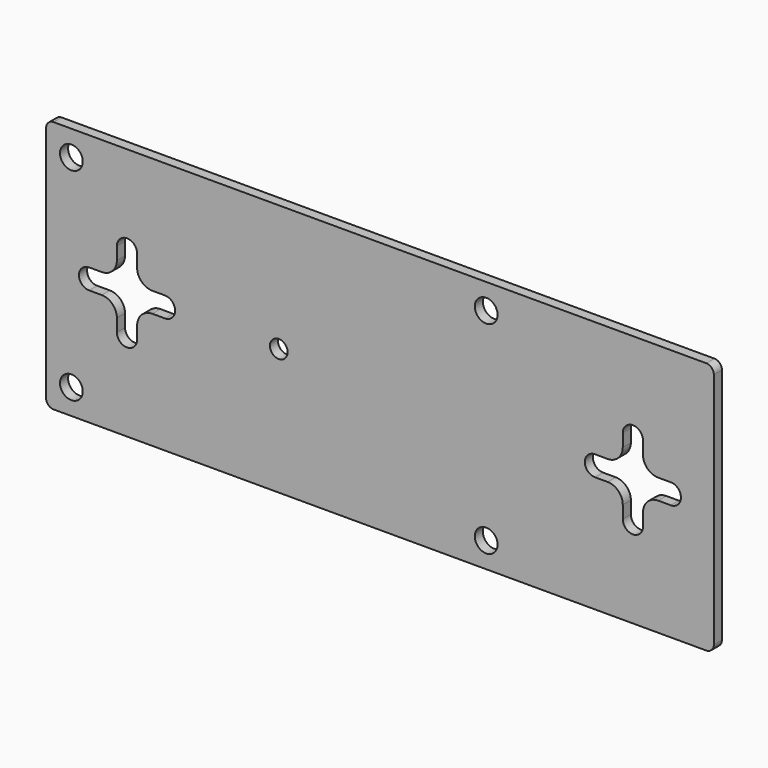
from build123d import *

# Parameters (mm, degrees)
F0_W     = 92
F0_H     = 50
F0_R     = 2.25
F0_R_2   = 1.75
F0_W_2   = 40
F1_DEPTH = 2
F2_R     = 3
F3_R     = 1.5


# Not quite as in the source:
# - a feature names something its author has since deleted; it is built from what else it names


with BuildPart() as f1:
    # F0 (on Front) → F1 (new body)
    with BuildSketch(Plane.XZ):
        with Locations((46, 25)):
            Rectangle(F0_W, F0_H)
        with Locations((5, 5)):
            Circle(F0_R, mode=Mode.SUBTRACT)
        with Locations((87, 5)):
            Circle(F0_R, mode=Mode.SUBTRACT)
        with BuildLine():
            Line((8.5, 27), (14, 27))
            Line((14, 27), (14, 32.5))
            ThreePointArc((14, 32.5), (16, 34.5), (18, 32.5))
            Line((18, 32.5), (18, 27))
            Line((18, 27), (23.5, 27))
            ThreePointArc((23.5, 27), (25.5, 25), (23.5, 23))
            Line((23.5, 23), (18, 23))
            Line((18, 23), (18, 17.5))
            ThreePointArc((18, 17.5), (16, 15.5), (14, 17.5))
            Line((14, 17.5), (14, 23))
            Line((14, 23), (8.5, 23))
            ThreePointArc((8.5, 23), (6.5, 25), (8.5, 27))
        make_face(mode=Mode.SUBTRACT)
        with Locations((46, 25)):
            Circle(F0_R_2, mode=Mode.SUBTRACT)
        with Locations((5, 45)):
            Circle(F0_R, mode=Mode.SUBTRACT)
        with Locations((87, 45)):
            Circle(F0_R, mode=Mode.SUBTRACT)
        with Locations((112, 25)):
            Rectangle(F0_W_2, F0_H)
        with BuildLine():
            Line((114, 27), (114, 32.5))
            ThreePointArc((114, 32.5), (116, 34.5), (118, 32.5))
            Line((118, 32.5), (118, 27))
            Line((118, 27), (123.5, 27))
            ThreePointArc((123.5, 27), (125.5, 25), (123.5, 23))
            Line((123.5, 23), (118, 23))
            Line((118, 23), (118, 17.5))
            ThreePointArc((118, 17.5), (116, 15.5), (114, 17.5))
            Line((114, 17.5), (114, 23))
            Line((114, 23), (108.5, 23))
            ThreePointArc((108.5, 23), (106.5, 25), (108.5, 27))
            Line((108.5, 27), (114, 27))
        make_face(mode=Mode.SUBTRACT)
    extrude(amount=F1_DEPTH)

    # F2
    f2_edges = [f1.edges().sort_by_distance(p)[0] for p in [
        (14, -1, 27),
        (14, -1, 23),
        (18, -1, 27),
        (18, -1, 23),
        (114, -1, 27),
        (118, -1, 27),
        (114, -1, 23),
        (118, -1, 23),
    ]]
    fillet(f2_edges, radius=F2_R)

    # F3
    f3_edges = [f1.edges().sort_by_distance(p)[0] for p in [
        (0, -1, 50),
        (0, -1, 0),
        (132, -1, 0),
        (132, -1, 50),
    ]]
    fillet(f3_edges, radius=F3_R)


solid = f1.part
